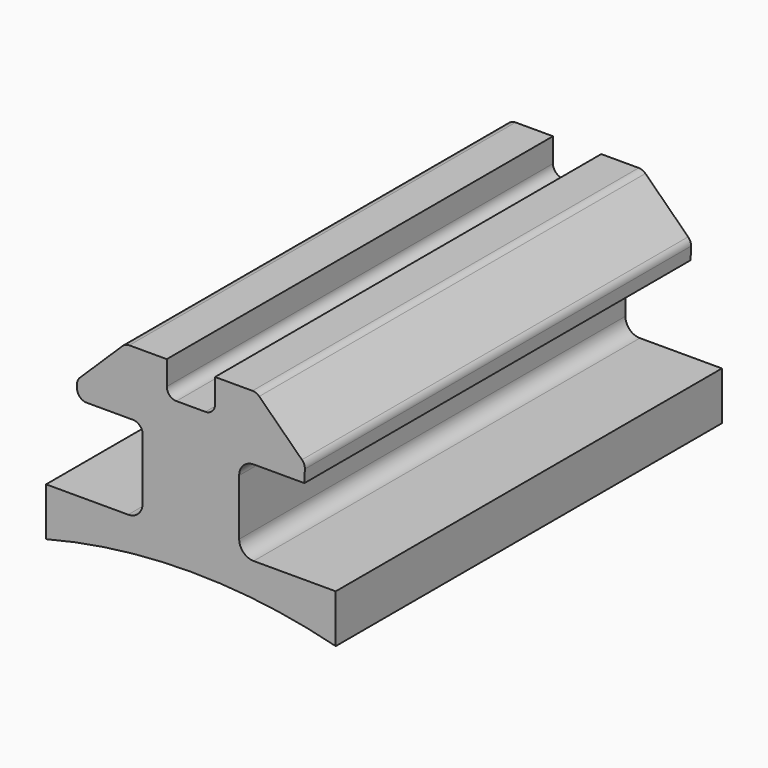
from build123d import *

# Parameters (mm, degrees)
F1_DEPTH = 10
F2_R     = 0.2
F3_R     = 0.3


# Not quite as in the source:
# - a feature names something its author has since deleted; it is built from what else it names


with BuildPart() as f1:
    # F0 (on Front) → F1 (new body)
    with BuildSketch(Plane.XZ):
        with BuildLine():
            Line((-3, 0.8663841993), (-3, -0.1336158007))
            ThreePointArc((-3, -0.1336158007), (-1.5120515098, 0.1517905158), (0, 0.2474341606))
            ThreePointArc((0, 0.2474341606), (1.5120515098, 0.1517905158), (3, -0.1336158007))
            Line((3, -0.1336158007), (3, 0.8663841993))
            Line((3, 0.8663841993), (1, 0.8663841993))
            Line((1, 0.8663841993), (1, 2.6280805469))
            Line((1, 2.6280805469), (2.3511576001, 2.6280805469))
            Line((2.3511576001, 2.6280805469), (2.363298554, 2.9764297366))
            Line((2.363298554, 2.9764297366), (1.357049332, 3.9621986704))
            Line((1.357049332, 3.9621986704), (0.5, 3.9621986704))
            Line((0.5, 3.9621986704), (0.5, 3.2621986704))
            Line((0.5, 3.2621986704), (0, 3.2621986704))
            Line((0, 3.2621986704), (-0.5, 3.2621986704))
            Line((-0.5, 3.2621986704), (-0.5, 3.9621986704))
            Line((-0.5, 3.9621986704), (-1.357049332, 3.9621986704))
            Line((-1.357049332, 3.9621986704), (-2.363298554, 2.9764297366))
            Line((-2.363298554, 2.9764297366), (-2.3511576001, 2.6280805469))
            Line((-2.3511576001, 2.6280805469), (-1, 2.6280805469))
            Line((-1, 2.6280805469), (-1, 0.8663841993))
            Line((-1, 0.8663841993), (-3, 0.8663841993))
        make_face()
    extrude(amount=F1_DEPTH)

    # F2
    f2_edges = [f1.edges().sort_by_distance(p)[0] for p in [
        (-0.5, -5, 3.262199),
        (0.5, -5, 3.262199),
        (2.363299, -5, 2.97643),
        (1.357049, -5, 3.962199),
        (-1, -5, 2.628081),
        (-2.351158, -5, 2.628081),
        (-2.363299, -5, 2.97643),
        (-1.357049, -5, 3.962199),
    ]]
    fillet(f2_edges, radius=F2_R)

    # F3
    f3_edges = [f1.edges().sort_by_distance(p)[0] for p in [
        (-1, -5, 0.866384),
        (1, -5, 0.866384),
        (1, -5, 2.628081),
    ]]
    fillet(f3_edges, radius=F3_R)


solid = f1.part
